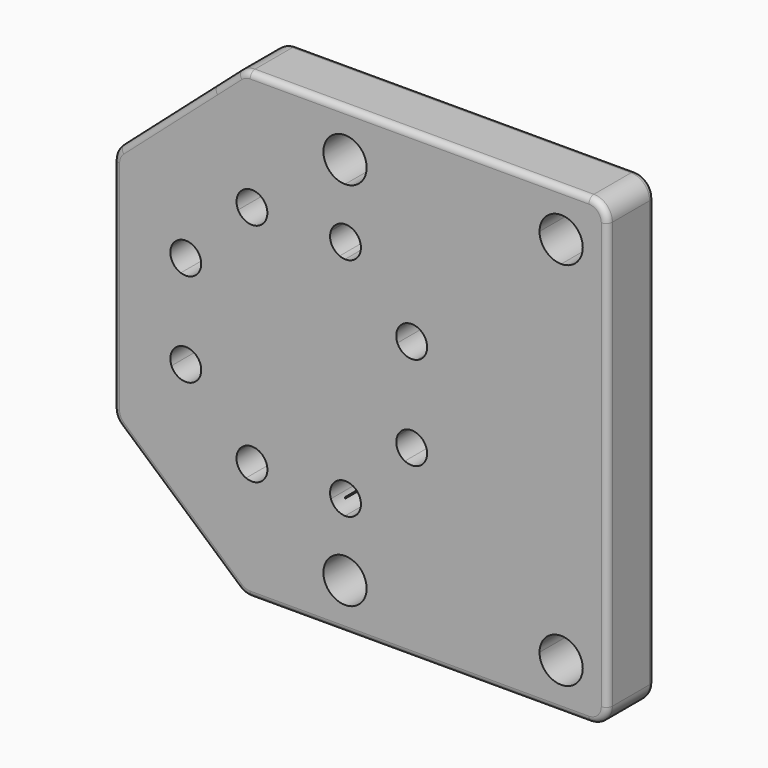
from build123d import *

# Parameters (mm, degrees)
F1_DEPTH = 9.525
F2_SIZE  = 2.2
F3_R     = 3
F4_R     = 1


# Not quite as in the source:
# - a feature names something its author has since deleted; it is built from what else it names


with BuildPart() as f1:
    # F0 (on Front) → F1 (new body)
    with BuildSketch(Plane.XZ):
        with BuildLine():
            ThreePointArc((-5.2116421806, 19.10180059), (0, 19.8), (5.2116421806, 19.10180059))
            ThreePointArc((5.2116421806, 19.10180059), (6.0920472722, 20.3039148078), (7.5, 20.7916245926))
            Line((7.5, 20.7916245926), (7.5, 26.5))
            ThreePointArc((7.5, 26.5), (5.0251262658, 32.4748737342), (11, 30))
            Line((11, 30), (12.4264068712, 30))
            Line((12.4264068712, 30), (15.533008589, 37.5))
            Line((15.533008589, 37.5), (-9, 37.5))
            Line((-9, 37.5), (-13.7864290327, 33.2833839474))
            Line((-13.7864290327, 33.2833839474), (-8.5338405417, 20.602513575))
            ThreePointArc((-8.5338405417, 20.602513575), (-6.547957057, 20.5711472518), (-5.2116421806, 19.10180059))
        make_face()
        with BuildLine():
            ThreePointArc((-17.1922002571, 9.8218252031), (-14.0007142675, 14.0007142675), (-9.8218252031, 17.1922002571))
            ThreePointArc((-9.8218252031, 17.1922002571), (-9.9158928806, 19.1761025564), (-8.5338405417, 20.602513575))
            Line((-8.5338405417, 20.602513575), (-13.7864290327, 33.2833839474))
            Line((-13.7864290327, 33.2833839474), (-30, 19))
            Line((-30, 19), (-30, 12.4264068712))
            Line((-30, 12.4264068712), (-20.602513575, 8.5338405417))
            ThreePointArc((-20.602513575, 8.5338405417), (-19.1761025564, 9.9158928806), (-17.1922002571, 9.8218252031))
        make_face()
        with BuildLine():
            Line((-15.9831159124, 6.6204233799), (0, 0))
            Line((0, 0), (-6.6204233799, 15.9831159124))
            ThreePointArc((-6.6204233799, 15.9831159124), (-8.4604197735, 15.9540538239), (-9.8218252031, 17.1922002571))
            ThreePointArc((-9.8218252031, 17.1922002571), (-14.0007142675, 14.0007142675), (-17.1922002571, 9.8218252031))
            ThreePointArc((-17.1922002571, 9.8218252031), (-16.171313363, 8.8997172669), (-15.7928147437, 7.5771319608))
            ThreePointArc((-15.7928147437, 7.5771319608), (-15.8408515427, 7.0894061558), (-15.9831159124, 6.6204233799))
        make_face()
        with BuildLine():
            Line((-6.6204233799, 15.9831159124), (0, 0))
            Line((0, 0), (6.6204233799, 15.9831159124))
            ThreePointArc((6.6204233799, 15.9831159124), (5.2987994528, 17.2636398399), (5.2116421806, 19.10180059))
            ThreePointArc((5.2116421806, 19.10180059), (0, 19.8), (-5.2116421806, 19.10180059))
            ThreePointArc((-5.2116421806, 19.10180059), (-5.1109887725, 18.7028608078), (-5.0771319608, 18.2928147437))
            ThreePointArc((-5.0771319608, 18.2928147437), (-5.4984579301, 16.9038891612), (-6.6204233799, 15.9831159124))
        make_face()
        with BuildLine():
            Line((7.5, 3.1066017178), (15.9831159124, 6.6204233799))
            ThreePointArc((15.9831159124, 6.6204233799), (15.9540538239, 8.4604197735), (17.1922002571, 9.8218252031))
            ThreePointArc((17.1922002571, 9.8218252031), (14.0007142675, 14.0007142675), (9.8218252031, 17.1922002571))
            ThreePointArc((9.8218252031, 17.1922002571), (8.8668288418, 16.1511607205), (7.5, 15.7940048949))
            Line((7.5, 15.7940048949), (7.5, 3.1066017178))
        make_face()
        with BuildLine():
            ThreePointArc((19.10180059, -5.2116421806), (19.6246739041, -2.6291013976), (19.8, 0))
            ThreePointArc((19.8, 0), (19.6246739041, 2.6291013976), (19.10180059, 5.2116421806))
            ThreePointArc((19.10180059, 5.2116421806), (17.2636398399, 5.2987994528), (15.9831159124, 6.6204233799))
            Line((15.9831159124, 6.6204233799), (7.5, 3.1066017178))
            Line((7.5, 3.1066017178), (7.5, -3.1066017178))
            Line((7.5, -3.1066017178), (15.9831159124, -6.6204233799))
            ThreePointArc((15.9831159124, -6.6204233799), (17.2636398399, -5.2987994528), (19.10180059, -5.2116421806))
        make_face()
        with BuildLine():
            ThreePointArc((17.1922002571, -9.8218252031), (15.9540538239, -8.4604197735), (15.9831159124, -6.6204233799))
            Line((15.9831159124, -6.6204233799), (7.5, -3.1066017178))
            Line((7.5, -3.1066017178), (7.5, -15.7940048949))
            ThreePointArc((7.5, -15.7940048949), (8.8668288418, -16.1511607205), (9.8218252031, -17.1922002571))
            ThreePointArc((9.8218252031, -17.1922002571), (14.0007142675, -14.0007142675), (17.1922002571, -9.8218252031))
        make_face()
        with BuildLine():
            ThreePointArc((20.602513575, -8.5338405417), (19.1761025564, -9.9158928806), (17.1922002571, -9.8218252031))
            ThreePointArc((17.1922002571, -9.8218252031), (14.0007142675, -14.0007142675), (9.8218252031, -17.1922002571))
            ThreePointArc((9.8218252031, -17.1922002571), (10.012469012, -17.7278957697), (10.0771319608, -18.2928147437))
            ThreePointArc((10.0771319608, -18.2928147437), (9.6558059916, -19.6817403263), (8.5338405417, -20.602513575))
            Line((8.5338405417, -20.602513575), (12.4264068712, -30))
            Line((12.4264068712, -30), (39, -30))
            ThreePointArc((39, -30), (40.0251262658, -27.5251262658), (42.5, -26.5))
            Line((42.5, -26.5), (42.5, -17.6040764009))
            Line((42.5, -17.6040764009), (20.602513575, -8.5338405417))
        make_face()
        with BuildLine():
            ThreePointArc((7.5, -20.7916245926), (6.0920472722, -20.3039148078), (5.2116421806, -19.10180059))
            ThreePointArc((5.2116421806, -19.10180059), (0, -19.8), (-5.2116421806, -19.10180059))
            ThreePointArc((-5.2116421806, -19.10180059), (-6.547957057, -20.5711472518), (-8.5338405417, -20.602513575))
            Line((-8.5338405417, -20.602513575), (-13.7864290327, -33.2833839474))
            Line((-13.7864290327, -33.2833839474), (-9, -37.5))
            Line((-9, -37.5), (15.533008589, -37.5))
            Line((15.533008589, -37.5), (12.4264068712, -30))
            Line((12.4264068712, -30), (11, -30))
            ThreePointArc((11, -30), (5.0251262658, -32.4748737342), (7.5, -26.5))
            Line((7.5, -26.5), (7.5, -20.7916245926))
        make_face()
        with BuildLine():
            Line((6.6204233799, -15.9831159124), (0, 0))
            Line((0, 0), (-6.6204233799, -15.9831159124))
            ThreePointArc((-6.6204233799, -15.9831159124), (-5.4984579301, -16.9038891612), (-5.0771319608, -18.2928147437))
            ThreePointArc((-5.0771319608, -18.2928147437), (-5.1109887725, -18.7028608078), (-5.2116421806, -19.10180059))
            ThreePointArc((-5.2116421806, -19.10180059), (0, -19.8), (5.2116421806, -19.10180059))
            ThreePointArc((5.2116421806, -19.10180059), (5.2987994528, -17.2636398399), (6.6204233799, -15.9831159124))
        make_face()
        with BuildLine():
            Line((-6.6204233799, -15.9831159124), (0, 0))
            Line((0, 0), (-15.9831159124, -6.6204233799))
            ThreePointArc((-15.9831159124, -6.6204233799), (-15.8408515427, -7.0894061558), (-15.7928147437, -7.5771319608))
            ThreePointArc((-15.7928147437, -7.5771319608), (-16.171313363, -8.8997172669), (-17.1922002571, -9.8218252031))
            ThreePointArc((-17.1922002571, -9.8218252031), (-14.0007142675, -14.0007142675), (-9.8218252031, -17.1922002571))
            ThreePointArc((-9.8218252031, -17.1922002571), (-8.4604197735, -15.9540538239), (-6.6204233799, -15.9831159124))
        make_face()
        with BuildLine():
            Line((-15.9831159124, -6.6204233799), (0, 0))
            Line((0, 0), (-15.9831159124, 6.6204233799))
            ThreePointArc((-15.9831159124, 6.6204233799), (-17.2636398399, 5.2987994528), (-19.10180059, 5.2116421806))
            ThreePointArc((-19.10180059, 5.2116421806), (-19.8, 0), (-19.10180059, -5.2116421806))
            ThreePointArc((-19.10180059, -5.2116421806), (-17.2636398399, -5.2987994528), (-15.9831159124, -6.6204233799))
        make_face()
        with BuildLine():
            ThreePointArc((-8.5338405417, -20.602513575), (-9.9158928806, -19.1761025564), (-9.8218252031, -17.1922002571))
            ThreePointArc((-9.8218252031, -17.1922002571), (-14.0007142675, -14.0007142675), (-17.1922002571, -9.8218252031))
            ThreePointArc((-17.1922002571, -9.8218252031), (-19.1761025564, -9.9158928806), (-20.602513575, -8.5338405417))
            Line((-20.602513575, -8.5338405417), (-30, -12.4264068712))
            Line((-30, -12.4264068712), (-30, -19))
            Line((-30, -19), (-13.7864290327, -33.2833839474))
            Line((-13.7864290327, -33.2833839474), (-8.5338405417, -20.602513575))
        make_face()
        with BuildLine():
            ThreePointArc((9.8218252031, 17.1922002571), (14.0007142675, 14.0007142675), (17.1922002571, 9.8218252031))
            ThreePointArc((17.1922002571, 9.8218252031), (19.1761025564, 9.9158928806), (20.602513575, 8.5338405417))
            Line((20.602513575, 8.5338405417), (42.5, 17.6040764009))
            Line((42.5, 17.6040764009), (42.5, 26.5))
            ThreePointArc((42.5, 26.5), (40.0251262658, 27.5251262658), (39, 30))
            Line((39, 30), (12.4264068712, 30))
            Line((12.4264068712, 30), (8.5338405417, 20.602513575))
            ThreePointArc((8.5338405417, 20.602513575), (9.6558059916, 19.6817403263), (10.0771319608, 18.2928147437))
            ThreePointArc((10.0771319608, 18.2928147437), (10.012469012, 17.7278957697), (9.8218252031, 17.1922002571))
        make_face()
        with BuildLine():
            Line((42.5, 26.5), (42.5, 17.6040764009))
            Line((42.5, 17.6040764009), (50, 20.7106781187))
            Line((50, 20.7106781187), (50, 37.5))
            Line((50, 37.5), (15.533008589, 37.5))
            Line((15.533008589, 37.5), (12.4264068712, 30))
            Line((12.4264068712, 30), (39, 30))
            ThreePointArc((39, 30), (42.5, 33.5), (46, 30))
            ThreePointArc((46, 30), (44.9748737342, 27.5251262658), (42.5, 26.5))
        make_face()
        with BuildLine():
            ThreePointArc((-20.602513575, -8.5338405417), (-20.5711472518, -6.547957057), (-19.10180059, -5.2116421806))
            ThreePointArc((-19.10180059, -5.2116421806), (-19.8, 0), (-19.10180059, 5.2116421806))
            ThreePointArc((-19.10180059, 5.2116421806), (-20.5711472518, 6.547957057), (-20.602513575, 8.5338405417))
            Line((-20.602513575, 8.5338405417), (-30, 12.4264068712))
            Line((-30, 12.4264068712), (-30, -12.4264068712))
            Line((-30, -12.4264068712), (-20.602513575, -8.5338405417))
        make_face()
        with BuildLine():
            ThreePointArc((19.10180059, 5.2116421806), (19.6246739041, 2.6291013976), (19.8, 0))
            ThreePointArc((19.8, 0), (19.6246739041, -2.6291013976), (19.10180059, -5.2116421806))
            ThreePointArc((19.10180059, -5.2116421806), (20.3265876681, -6.1232517415), (20.7928147437, -7.5771319608))
            ThreePointArc((20.7928147437, -7.5771319608), (20.7447779447, -8.0648577659), (20.602513575, -8.5338405417))
            Line((20.602513575, -8.5338405417), (42.5, -17.6040764009))
            Line((42.5, -17.6040764009), (42.5, 17.6040764009))
            Line((42.5, 17.6040764009), (20.602513575, 8.5338405417))
            ThreePointArc((20.602513575, 8.5338405417), (20.7447779447, 8.0648577659), (20.7928147437, 7.5771319608))
            ThreePointArc((20.7928147437, 7.5771319608), (20.3265876681, 6.1232517415), (19.10180059, 5.2116421806))
        make_face()
        Polygon((50, 20.7106781187), (42.5, 17.6040764009), (42.5, -17.6040764009), (50, -20.7106781187), align=None)
        with BuildLine():
            Line((50, -20.7106781187), (42.5, -17.6040764009))
            Line((42.5, -17.6040764009), (42.5, -26.5))
            ThreePointArc((42.5, -26.5), (44.9748737342, -27.5251262658), (46, -30))
            ThreePointArc((46, -30), (42.5, -33.5), (39, -30))
            Line((39, -30), (12.4264068712, -30))
            Line((12.4264068712, -30), (15.533008589, -37.5))
            Line((15.533008589, -37.5), (50, -37.5))
            Line((50, -37.5), (50, -20.7106781187))
        make_face()
        with BuildLine():
            Line((7.5, -15.7940048949), (7.5, -3.1066017178))
            Line((7.5, -3.1066017178), (0, 0))
            Line((0, 0), (6.6204233799, -15.9831159124))
            ThreePointArc((6.6204233799, -15.9831159124), (7.0516347575, -15.8486681259), (7.5, -15.7940048949))
        make_face()
        Polygon((7.5, -3.1066017178), (7.5, 3.1066017178), (0, 0), align=None)
        with BuildLine():
            Line((0, 0), (7.5, 3.1066017178))
            Line((7.5, 3.1066017178), (7.5, 15.7940048949))
            ThreePointArc((7.5, 15.7940048949), (7.0516347575, 15.8486681259), (6.6204233799, 15.9831159124))
            Line((6.6204233799, 15.9831159124), (0, 0))
        make_face()
        with BuildLine():
            Line((12.4264068712, -30), (8.5338405417, -20.602513575))
            ThreePointArc((8.5338405417, -20.602513575), (8.0269702672, -20.7520108518), (7.5, -20.7916245926))
            Line((7.5, -20.7916245926), (7.5, -26.5))
            ThreePointArc((7.5, -26.5), (9.9748737342, -27.5251262658), (11, -30))
            Line((11, -30), (12.4264068712, -30))
        make_face()
        with BuildLine():
            ThreePointArc((7.5, 20.7916245926), (8.0269702672, 20.7520108518), (8.5338405417, 20.602513575))
            Line((8.5338405417, 20.602513575), (12.4264068712, 30))
            Line((12.4264068712, 30), (11, 30))
            ThreePointArc((11, 30), (9.9748737342, 27.5251262658), (7.5, 26.5))
            Line((7.5, 26.5), (7.5, 20.7916245926))
        make_face()
    extrude(amount=F1_DEPTH)

    # F2
    f2_edges = [f1.edges().sort_by_distance(p)[0] for p in [
        (7.654264, 0, 15.794005),
        (-9.942622, 0, 17.483829),
        (-17.483829, 0, 9.942622),
        (-15.983116, 0, -6.620423),
        (-6.620423, 0, -15.983116),
        (6.620423, 0, -15.983116),
        (17.483829, 0, -9.942622),
        (15.983116, 0, 6.620423),
    ]]
    chamfer(f2_edges, length=F2_SIZE)

    # F3
    f3_edges = [f1.edges().sort_by_distance(p)[0] for p in [
        (50, -4.7625, 37.5),
        (50, -4.7625, -37.5),
        (-9, -4.7625, -37.5),
        (-9, -4.7625, 37.5),
        (-30, -4.7625, 19),
        (-30, -4.7625, -19),
    ]]
    fillet(f3_edges, radius=F3_R)

    # F4
    f4_edges = [f1.edges().sort_by_distance(p)[0] for p in [
        (19.566481, -9.525, 37.5),
        (-30, -9.525, 0),
        (19.566481, -9.525, -37.5),
        (50, -9.525, 0),
        (50, 0, 0),
        (19.566481, 0, 37.5),
        (-30, 0, 0),
        (19.566481, 0, -37.5),
        (49.12132, -9.525, 36.62132),
        (49.12132, 0, 36.62132),
        (49.12132, -9.525, -36.62132),
        (49.12132, 0, -36.62132),
        (-8.926936, -9.525, -37.306531),
        (-19.41661, -9.525, -28.323462),
        (-29.733978, -9.525, -18.879827),
        (-29.733978, -9.525, 18.879827),
        (-8.926936, -9.525, 37.306531),
        (-19.41661, -9.525, 28.323462),
        (-8.926936, 0, -37.306531),
        (-19.41661, 0, -28.323462),
        (-29.733978, 0, -18.879827),
        (-29.733978, 0, 18.879827),
        (-8.926936, 0, 37.306531),
        (-19.41661, 0, 28.323462),
    ]]
    fillet(f4_edges, radius=F4_R)


with BuildPart() as f1b:
    # F0 (on Front) → F1, piece 2 (new body)
    with BuildSketch(Plane.XZ):
        with BuildLine():
            ThreePointArc((7.5, -18.3245736649), (7.5385827049, -18.3087348225), (7.5771319608, -18.2928147437))
            Line((7.5771319608, -18.2928147437), (7.5, -18.1066017178))
            Line((7.5, -18.1066017178), (7.5, -18.3245736649))
        make_face()
    extrude(amount=F1_DEPTH)


solid = Compound([f1.part, f1b.part])
